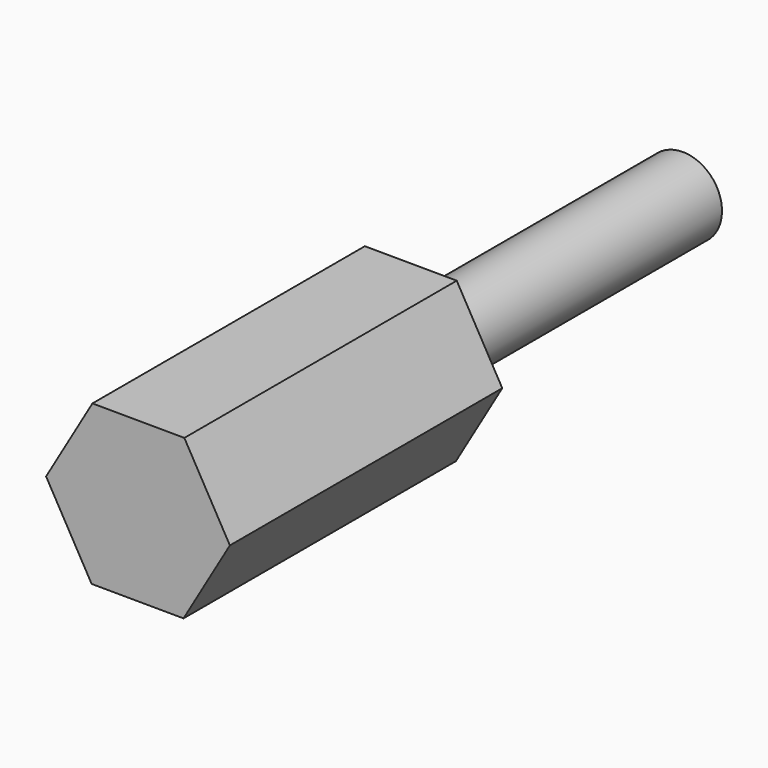
from build123d import *

# Parameters (mm, degrees)
F1_DEPTH = 254
F4_R     = 29.2765375906
F5_DEPTH = 254


# Not quite as in the source:
# - the program builds the solid bodies; features that only make, move or delete a surface that nothing else refers to are left out


with BuildPart() as f1:
    # F0 (on Front) → F1 (new body)
    with BuildSketch(Plane.XZ):
        Polygon((33.9669666181, -59.5514180462), (68.5565241684, -0.3594530423), (34.5895575503, 59.1919650039), (-33.9669666181, 59.5514180462), (-68.5565241684, 0.3594530423), (-34.5895575503, -59.1919650039), align=None)
    extrude(amount=F1_DEPTH)

    # F4 (on face) → F5 (join)
    with BuildSketch(Plane(origin=(0, 0, 0), x_dir=(-1, 0, 0), z_dir=(0, 1, 0))):
        Circle(F4_R)
    extrude(amount=F5_DEPTH)


solid = f1.part
